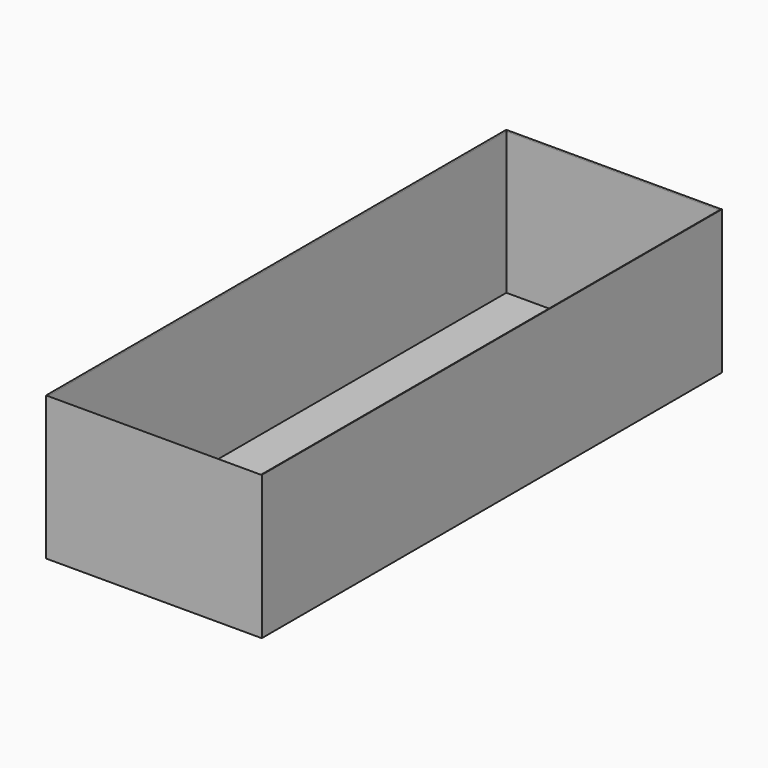
from build123d import *

# Parameters (mm, degrees)
F0_W         = 914.4
F0_H         = 2438.4
F1_DEPTH     = 609.6
F3_T         = -2.54
F4_T1_DEPTH  = 2433.32
F4_T3_DEPTH  = 909.32
F4_T9_DEPTH  = 2446.02
F4_T15_DEPTH = 922.02
F4_T24_DEPTH = 2446.02
F4_T30_DEPTH = 922.02


# Not quite as in the source:
# - a fillet or chamfer that OpenCascade refuses, or shapes differently, is made with other operations: its cross-section is extruded or revolved along the edge and cut away or added


with BuildPart() as f1:
    # F0 (on Top) → F1 (new body)
    with BuildSketch(Plane.XY):
        with Locations((-243.063261795, 394.9879257202)):
            Rectangle(F0_W, F0_H)
    extrude(amount=F1_DEPTH)

    # F3
    f3_openings = [f1.faces().sort_by_distance(p)[0] for p in [
        (-243.063262, 394.987926, 609.6),
    ]]
    offset(amount=F3_T, openings=f3_openings)

    # F4: fillet of radius 5.08 on 3 edges, made by hand

    # F4_s2 → F4_t1 (cut)
    with BuildSketch(Plane.XZ.offset(-1611.6479257202)):
        with BuildLine():
            ThreePointArc((-702.803261795, 609.6), (-699.2111593466, 608.1121024484), (-697.723261795, 604.52))
            Line((-697.723261795, 604.52), (-697.723261795, 609.6))
            Line((-697.723261795, 609.6), (-702.803261795, 609.6))
        make_face()
    extrude(amount=F4_T1_DEPTH, mode=Mode.SUBTRACT)

    # F4_s4 → F4_t3 (cut)
    with BuildSketch(Plane.YZ.offset(-697.723261795)):
        with BuildLine():
            ThreePointArc((-826.7520742798, 609.6), (-823.1599718314, 608.1121024484), (-821.6720742798, 604.52))
            Line((-821.6720742798, 604.52), (-821.6720742798, 609.6))
            Line((-821.6720742798, 609.6), (-826.7520742798, 609.6))
        make_face()
        with BuildLine():
            ThreePointArc((1616.7279257202, 609.6), (1613.1358232718, 608.1121024484), (1611.6479257202, 604.52))
            Line((1611.6479257202, 604.52), (1611.6479257202, 609.6))
            Line((1611.6479257202, 609.6), (1616.7279257202, 609.6))
        make_face()
    extrude(amount=F4_T3_DEPTH, mode=Mode.SUBTRACT)


with BuildPart() as f4_tool7:
    # F4_s8 → F4_t9 (new body)
    with BuildSketch(Plane.XZ.offset(-1624.3479257202)):
        with BuildLine():
            ThreePointArc((-702.803261795, 609.6), (-699.2111593466, 608.1121024484), (-697.723261795, 604.52))
            Line((-697.723261795, 604.52), (-697.723261795, 609.6))
            Line((-697.723261795, 609.6), (-702.803261795, 609.6))
        make_face()
    extrude(amount=F4_T9_DEPTH)

    split(bisect_by=Plane.YZ.offset(-700.263261795), keep=Keep.TOP)

    split(bisect_by=Plane.XZ.offset(-1614.1879257202), keep=Keep.TOP)

    split(bisect_by=Plane.XZ.offset(-1611.6479257202), keep=Keep.BOTTOM)


with BuildPart() as f4_tool13:
    # F4_s14 → F4_t15 (new body)
    with BuildSketch(Plane.YZ.offset(211.596738205)):
        with BuildLine():
            ThreePointArc((1616.7279257202, 609.6), (1613.1358232718, 608.1121024484), (1611.6479257202, 604.52))
            Line((1611.6479257202, 604.52), (1611.6479257202, 609.6))
            Line((1611.6479257202, 609.6), (1616.7279257202, 609.6))
        make_face()
    extrude(amount=-F4_T15_DEPTH)

    split(bisect_by=Plane.YZ.offset(-700.263261795), keep=Keep.TOP)

    split(bisect_by=Plane.XZ.offset(-1614.1879257202), keep=Keep.TOP)

    split(bisect_by=Plane.YZ.offset(-697.723261795), keep=Keep.BOTTOM)


with BuildPart() as f4_tool7_1:
    add(f4_tool7.part)

    # F4_t19: intersect F4_tool13
    add(f4_tool13.part, mode=Mode.INTERSECT)


with BuildPart() as f1_1:
    add(f1.part)

    # F4_t5: cut F4_tool7
    add(f4_tool7_1.part, mode=Mode.SUBTRACT)


with BuildPart() as f4_tool22:
    # F4_s23 → F4_t24 (new body)
    with BuildSketch(Plane.XZ.offset(-1611.6479257202)):
        with BuildLine():
            ThreePointArc((-702.803261795, 609.6), (-699.2111593466, 608.1121024484), (-697.723261795, 604.52))
            Line((-697.723261795, 604.52), (-697.723261795, 609.6))
            Line((-697.723261795, 609.6), (-702.803261795, 609.6))
        make_face()
    extrude(amount=F4_T24_DEPTH)

    split(bisect_by=Plane.YZ.offset(-700.263261795), keep=Keep.TOP)

    split(bisect_by=Plane.XZ.offset(824.2120742798), keep=Keep.BOTTOM)

    split(bisect_by=Plane.XZ.offset(821.6720742798), keep=Keep.TOP)


with BuildPart() as f4_tool28:
    # F4_s29 → F4_t30 (new body)
    with BuildSketch(Plane.YZ.offset(-710.423261795)):
        with BuildLine():
            ThreePointArc((-826.7520742798, 609.6), (-823.1599718314, 608.1121024484), (-821.6720742798, 604.52))
            Line((-821.6720742798, 604.52), (-821.6720742798, 609.6))
            Line((-821.6720742798, 609.6), (-826.7520742798, 609.6))
        make_face()
    extrude(amount=F4_T30_DEPTH)

    split(bisect_by=Plane.YZ.offset(-700.263261795), keep=Keep.TOP)

    split(bisect_by=Plane.XZ.offset(824.2120742798), keep=Keep.BOTTOM)

    split(bisect_by=Plane.YZ.offset(-697.723261795), keep=Keep.BOTTOM)


with BuildPart() as f4_tool22_1:
    add(f4_tool22.part)

    # F4_t34: intersect F4_tool28
    add(f4_tool28.part, mode=Mode.INTERSECT)


with BuildPart() as f1_2:
    add(f1_1.part)

    # F4_t20: cut F4_tool22
    add(f4_tool22_1.part, mode=Mode.SUBTRACT)


solid = f1_2.part
